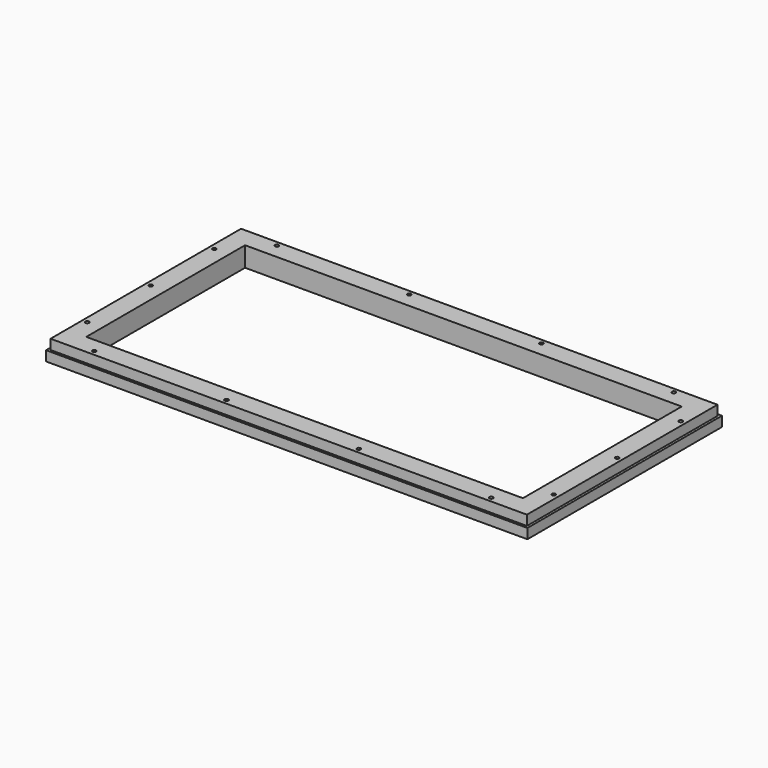
from build123d import *

# Parameters (mm, degrees)
F0_W     = 609.6
F0_H     = 304.8
F0_W_2   = 558.7999820709
F0_H_2   = 253.9999820709
F1_DEPTH = 25.4
F2_W     = 609.6
F2_H     = 304.8
F2_W_2   = 584.2
F2_H_2   = 279.4
F3_DEPTH = 3.175
F4_W     = 615.95
F4_H     = 311.15
F4_W_2   = 590.55
F4_H_2   = 285.75
F5_DEPTH = 3.175
F6_W     = 615.95
F6_H     = 311.15
F6_W_2   = 609.6
F6_H_2   = 304.8
F7_DEPTH = 9.525
F8_R     = 2.38125
F9_DEPTH = 25.401


with BuildPart() as f1:
    # F0 (on Top) → F1 (new body)
    with BuildSketch(Plane.XY):
        Rectangle(F0_W, F0_H)
        Rectangle(F0_W_2, F0_H_2, mode=Mode.SUBTRACT)
    extrude(amount=F1_DEPTH)

    # F2 (on Top) → F3 (cut)
    with BuildSketch(Plane.XY):
        Rectangle(F2_W, F2_H)
        Rectangle(F2_W_2, F2_H_2, mode=Mode.SUBTRACT)
    extrude(amount=F3_DEPTH, mode=Mode.SUBTRACT)


with BuildPart() as f5:
    # F4 (on Top) → F5 (new body)
    with BuildSketch(Plane.XY):
        Rectangle(F4_W, F4_H)
        Rectangle(F4_W_2, F4_H_2, mode=Mode.SUBTRACT)
    extrude(amount=F5_DEPTH)

    # F6 (on face) → F7 (join)
    with BuildSketch(Plane.XY.offset(3.175)):
        Rectangle(F6_W, F6_H)
        Rectangle(F6_W_2, F6_H_2, mode=Mode.SUBTRACT)
    extrude(amount=F7_DEPTH)


with BuildPart() as f9_tool:
    # F8 (on Top) → F9 (new body, through all)
    with BuildSketch(Plane.XY):
        with Locations((-253.9999910355, 146.05)):
            Circle(F8_R)
        with Locations((-84.6666636785, 146.05)):
            Circle(F8_R)
        with Locations((84.6666636785, 146.05)):
            Circle(F8_R)
        with Locations((253.9999910355, 146.05)):
            Circle(F8_R)
        with Locations((298.45, 101.5999910355)):
            Circle(F8_R)
        with Locations((298.45, 0)):
            Circle(F8_R)
        with Locations((298.45, -101.5999910355)):
            Circle(F8_R)
        with Locations((253.9999910355, -146.05)):
            Circle(F8_R)
        with Locations((84.6666636785, -146.05)):
            Circle(F8_R)
        with Locations((-84.6666636785, -146.05)):
            Circle(F8_R)
        with Locations((-253.9999910355, -146.05)):
            Circle(F8_R)
        with Locations((-298.45, 101.5999910355)):
            Circle(F8_R)
        with Locations((-298.45, 0)):
            Circle(F8_R)
        with Locations((-298.45, -101.5999910355)):
            Circle(F8_R)
    extrude(amount=F9_DEPTH)


with BuildPart() as f1_1:
    add(f1.part)

    # F9: cut by f9_tool
    add(f9_tool.part, mode=Mode.SUBTRACT)


with BuildPart() as f5_1:
    add(f5.part)

    # F9: cut by f9_tool
    add(f9_tool.part, mode=Mode.SUBTRACT)


solid = Compound([f1_1.part, f5_1.part])
